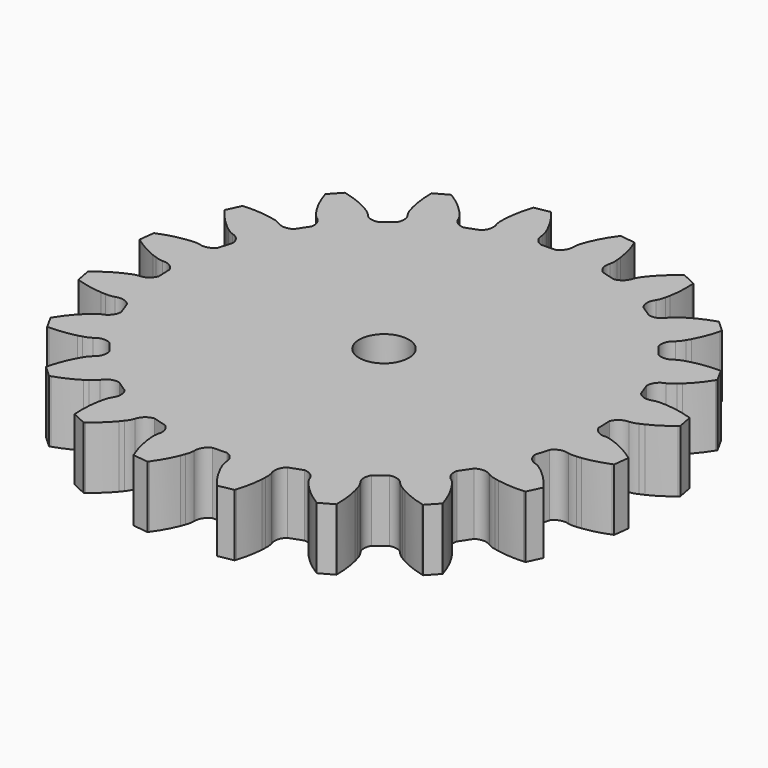
from build123d import *

# Parameters (mm, degrees)
F0_R     = 2
F1_DEPTH = 5


# Not quite as in the source:
# - ends of sketch curves that miss each other by under 0.0002 mm in the source are joined


with BuildPart() as f1:
    # F0 (on Top) → F1 (new body)
    with BuildSketch(Plane.XY):
        with BuildLine():
            ThreePointArc((6.2795421224, 17.2528949711), (5.9372089952, 16.6897816616), (5.3292660269, 16.4354316735))
            Line((5.3292660269, 16.4354316735), (4.238829, 16.749832))
            ThreePointArc((4.238829, 16.749832), (3.8596188728, 17.2887997141), (3.8696296081, 17.947730134))
            ThreePointArc((3.8696296081, 17.947730134), (3.9098326338, 18.2899811197), (3.8900979523, 18.6340169931))
            Line((3.8900979523, 18.6340169931), (3.85527, 18.998924))
            ThreePointArc((3.85527, 18.998924), (3.6466807278, 20.0297301014), (3.312523712, 21.0269318832))
            Line((3.312523712, 21.0269318832), (3.259754, 21.158733))
            Line((3.259754, 21.158733), (2.017975, 21.313043))
            Line((2.017975, 21.313043), (1.934553, 21.198166))
            ThreePointArc((1.934553, 21.198166), (1.3664960287, 20.3130778427), (0.9119624977, 19.3646732036))
            Line((0.9119624977, 19.3646732036), (0.78888, 19.019387))
            ThreePointArc((0.78888, 19.019387), (0.6855432602, 18.6906435099), (0.6407608463, 18.3489640066))
            ThreePointArc((0.6407608463, 18.3489640066), (0.4891935662, 17.707625921), (-0.0103961103, 17.2778602637))
            Line((-0.0103961103, 17.2778602637), (-1.144616, 17.239907))
            ThreePointArc((-1.144616, 17.239907), (-1.6718177114, 17.6353149503), (-1.8659179767, 18.2650879996))
            ThreePointArc((-1.8659179767, 18.2650879996), (-1.9334407464, 18.6030096473), (-2.0585228, 18.9241090987))
            Line((-2.0585228, 18.9241090987), (-2.204412, 19.260394))
            ThreePointArc((-2.204412, 19.260394), (-2.7213270618, 20.1762961465), (-3.3472816933, 21.021431258))
            Line((-3.3472816933, 21.021431258), (-3.438197, 21.130471))
            Line((-3.438197, 21.130471), (-4.666884, 20.893497))
            Line((-4.666884, 20.893497), (-4.710725, 20.758465))
            ThreePointArc((-4.710725, 20.758465), (-4.9774723389, 19.7411552057), (-5.1166863028, 18.6987100215))
            Line((-5.1166863028, 18.6987100215), (-5.127045, 18.332291))
            ThreePointArc((-5.127045, 18.332291), (-5.1237362452, 17.9877011205), (-5.0607420433, 17.648905988))
            ThreePointArc((-5.0607420433, 17.648905988), (-5.0067049946, 16.9921224763), (-5.3490383291, 16.4290093826))
            Line((-5.3490383291, 16.4290093826), (-6.416021, 16.04242))
            ThreePointArc((-6.416021, 16.04242), (-7.0396053696, 16.2555600272), (-7.4188161099, 16.7945296579))
            ThreePointArc((-7.4188161099, 16.7945296579), (-7.5874575289, 17.0950469339), (-7.805642719, 17.361778299))
            Line((-7.805642719, 17.361778299), (-8.04831, 17.636525))
            ThreePointArc((-8.04831, 17.636525), (-8.822951725, 18.3478589308), (-9.6794307515, 18.9581993988))
            Line((-9.6794307515, 18.9581993988), (-9.799595, 19.033811))
            Line((-9.799595, 19.033811), (-10.894916, 18.428749))
            Line((-10.894916, 18.428749), (-10.894883, 18.286778))
            ThreePointArc((-10.894883, 18.286778), (-10.8342091412, 17.2368317381), (-10.6444761882, 16.2023879533))
            Line((-10.6444761882, 16.2023879533), (-10.541097, 15.850697))
            ThreePointArc((-10.541097, 15.850697), (-10.4314703301, 15.5240012928), (-10.2668657315, 15.2212541779))
            ThreePointArc((-10.2668657315, 15.2212541779), (-10.0125146027, 14.6133081664), (-10.1640812817, 13.9719691712))
            Line((-10.1640812817, 13.9719691712), (-11.059377, 13.274587))
            ThreePointArc((-11.059377, 13.274587), (-11.7183065515, 13.284596409), (-12.2455078303, 13.6800041194))
            ThreePointArc((-12.2455078303, 13.6800041194), (-12.4987620125, 13.9137031189), (-12.7886931291, 14.0999567544))
            Line((-12.7886931291, 14.0999567544), (-13.104382, 14.286265))
            ThreePointArc((-13.104382, 14.286265), (-14.0609263803, 14.723407966), (-15.0640920585, 15.0392097641))
            Line((-15.0640920585, 15.0392097641), (-15.20174, 15.073991))
            Line((-15.20174, 15.073991), (-16.056476, 14.16007))
            Line((-16.056476, 14.16007), (-16.012575, 14.025056))
            ThreePointArc((-16.012575, 14.025056), (-15.6304195227, 13.0452436642), (-15.1303121532, 12.1200599045))
            Line((-15.1303121532, 12.1200599045), (-14.923314, 11.817531))
            ThreePointArc((-14.923314, 11.817531), (-14.7180959918, 11.5407024212), (-14.4679937608, 11.303638301))
            ThreePointArc((-14.4679937608, 11.303638301), (-14.0382262447, 10.8040458442), (-13.9841899305, 10.1472587473))
            Line((-13.9841899305, 10.1472587473), (-14.620166, 9.207347))
            ThreePointArc((-14.620166, 9.207347), (-15.2499383725, 9.0132480289), (-15.87352412, 9.22638884))
            ThreePointArc((-15.87352412, 9.22638884), (-16.1865976161, 9.3703858687), (-16.5198940041, 9.4579299761))
            Line((-16.5198940041, 9.4579299761), (-16.877707, 9.537571))
            ThreePointArc((-16.877707, 9.537571), (-17.9225197597, 9.657729375), (-18.9741749647, 9.6480795034))
            Line((-18.9741749647, 9.6480795034), (-19.115832, 9.638622))
            Line((-19.115832, 9.638622), (-19.646318, 8.5053))
            Line((-19.646318, 8.5053), (-19.562844, 8.390465))
            ThreePointArc((-19.562844, 8.390465), (-18.8966142395, 7.5766989313), (-18.1350863391, 6.8513385968))
            Line((-18.1350863391, 6.8513385968), (-17.844734, 6.627582))
            ThreePointArc((-17.844734, 6.627582), (-17.5640125021, 6.4277153406), (-17.2528940551, 6.2795398526))
            ThreePointArc((-17.2528940551, 6.2795398526), (-16.6897826616, 5.9372089952), (-16.4354326735, 5.3292660269))
            Line((-16.4354326735, 5.3292660269), (-16.74983, 4.238829))
            ThreePointArc((-16.74983, 4.238829), (-17.2888002619, 3.8596190122), (-17.9477302386, 3.869629302))
            ThreePointArc((-17.9477302386, 3.869629302), (-18.2899776143, 3.9098326485), (-18.6340139723, 3.8900978098))
            Line((-18.6340139723, 3.8900978098), (-18.998923, 3.85527))
            ThreePointArc((-18.998923, 3.85527), (-20.0297311014, 3.6466807278), (-21.0269328832, 3.312523712))
            Line((-21.0269328832, 3.312523712), (-21.158733, 3.259754))
            Line((-21.158733, 3.259754), (-21.313042, 2.017975))
            Line((-21.313042, 2.017975), (-21.198166, 1.934553))
            ThreePointArc((-21.198166, 1.934553), (-20.3130761949, 1.3664962251), (-19.3646712036, 0.9119624977))
            Line((-19.3646712036, 0.9119624977), (-19.019386, 0.78888))
            ThreePointArc((-19.019386, 0.78888), (-18.6906425099, 0.6855432602), (-18.3489630066, 0.6407608463))
            ThreePointArc((-18.3489630066, 0.6407608463), (-17.7076245117, 0.4891939253), (-17.2778584127, -0.0103957543))
            Line((-17.2778584127, -0.0103957543), (-17.239905, -1.144616))
            ThreePointArc((-17.239905, -1.144616), (-17.6353134914, -1.6718180921), (-18.2650869994, -1.8659179615))
            ThreePointArc((-18.2650869994, -1.8659179615), (-18.6030081703, -1.933440607), (-18.9241080987, -2.0585228))
            Line((-18.9241080987, -2.0585228), (-19.260395, -2.204412))
            ThreePointArc((-19.260395, -2.204412), (-20.1762931465, -2.7213270618), (-21.021428258, -3.3472816933))
            Line((-21.021428258, -3.3472816933), (-21.130471, -3.438197))
            Line((-21.130471, -3.438197), (-20.893497, -4.666884))
            Line((-20.893497, -4.666884), (-20.758464, -4.710725))
            ThreePointArc((-20.758464, -4.710725), (-19.7411532504, -4.9774725271), (-18.6987080265, -5.1166863735))
            Line((-18.6987080265, -5.1166863735), (-18.332287, -5.127045))
            ThreePointArc((-18.332287, -5.127045), (-17.9877021205, -5.1237362452), (-17.648906988, -5.0607420433))
            ThreePointArc((-17.648906988, -5.0607420433), (-16.9921192426, -5.0067048135), (-16.4290058079, -5.3490378347))
            Line((-16.4290058079, -5.3490378347), (-16.042417, -6.416021))
            ThreePointArc((-16.042417, -6.416021), (-16.2555580318, -7.0396053757), (-16.7945276579, -7.4188161099))
            ThreePointArc((-16.7945276579, -7.4188161099), (-17.0950436381, -7.5874573272), (-17.3617747863, -7.8056422191))
            Line((-17.3617747863, -7.8056422191), (-17.636522, -8.04831))
            ThreePointArc((-17.636522, -8.04831), (-18.3478589308, -8.822951725), (-18.9581993988, -9.6794307515))
            Line((-18.9581993988, -9.6794307515), (-19.03381, -9.799595))
            Line((-19.03381, -9.799595), (-18.42875, -10.894916))
            Line((-18.42875, -10.894916), (-18.286777, -10.894883))
            ThreePointArc((-18.286777, -10.894883), (-17.2368287381, -10.8342091412), (-16.2023849533, -10.6444761882))
            Line((-16.2023849533, -10.6444761882), (-15.850698, -10.541097))
            ThreePointArc((-15.850698, -10.541097), (-15.5239982928, -10.4314703301), (-15.2212511779, -10.2668657315))
            ThreePointArc((-15.2212511779, -10.2668657315), (-14.61330897, -10.0125146688), (-13.9719699014, -10.1640808378))
            Line((-13.9719699014, -10.1640808378), (-13.274586, -11.059377))
            ThreePointArc((-13.274586, -11.059377), (-13.2845965413, -11.7183069384), (-13.6800047882, -12.245508301))
            ThreePointArc((-13.6800047882, -12.245508301), (-13.9137001189, -12.4987620125), (-14.0999537544, -12.7886931291))
            Line((-14.0999537544, -12.7886931291), (-14.286265, -13.104382))
            ThreePointArc((-14.286265, -13.104382), (-14.723406966, -14.0609263803), (-15.0392087641, -15.0640920585))
            Line((-15.0392087641, -15.0640920585), (-15.073988, -15.20174))
            Line((-15.073988, -15.20174), (-14.160067, -16.056476))
            Line((-14.160067, -16.056476), (-14.025055, -16.012575))
            ThreePointArc((-14.025055, -16.012575), (-13.0452438471, -15.6304191443), (-12.1200601843, -15.1303117043))
            Line((-12.1200601843, -15.1303117043), (-11.81753, -14.923314))
            ThreePointArc((-11.81753, -14.923314), (-11.5406986541, -14.7180961981), (-11.3036346881, -14.4679942479))
            ThreePointArc((-11.3036346881, -14.4679942479), (-10.8040460838, -14.038226345), (-10.1472587473, -13.9841899305))
            Line((-10.1472587473, -13.9841899305), (-9.207345, -14.620166))
            ThreePointArc((-9.207345, -14.620166), (-9.0132460291, -15.2499383848), (-9.2263872, -15.8735246))
            ThreePointArc((-9.2263872, -15.8735246), (-9.3703848687, -16.1865976161), (-9.4579289761, -16.5198940041))
            Line((-9.4579289761, -16.5198940041), (-9.537568, -16.877707))
            ThreePointArc((-9.537568, -16.877707), (-9.6577283769, -17.9225197951), (-9.6480784984, -18.9741750354))
            Line((-9.6480784984, -18.9741750354), (-9.638618, -19.115832))
            Line((-9.638618, -19.115832), (-8.505301, -19.646318))
            Line((-8.505301, -19.646318), (-8.390464, -19.562844))
            ThreePointArc((-8.390464, -19.562844), (-7.5766996953, -18.8966140207), (-6.8513391825, -18.1350858465))
            Line((-6.8513391825, -18.1350858465), (-6.62758, -17.844734))
            ThreePointArc((-6.62758, -17.844734), (-6.4277133406, -17.5640125021), (-6.2795378526, -17.2528940551))
            ThreePointArc((-6.2795378526, -17.2528940551), (-5.9372079952, -16.6897826616), (-5.3292650269, -16.4354326735))
            Line((-5.3292650269, -16.4354326735), (-4.238828, -16.74983))
            ThreePointArc((-4.238828, -16.74983), (-3.859617942, -17.2888004896), (-3.8696281974, -17.9477299325))
            ThreePointArc((-3.8696281974, -17.9477299325), (-3.9098316455, -18.289977513), (-3.8900968098, -18.6340139723))
            Line((-3.8900968098, -18.6340139723), (-3.855269, -18.998923))
            ThreePointArc((-3.855269, -18.998923), (-3.6466796615, -20.0297313492), (-3.3125225708, -21.0269332314))
            Line((-3.3125225708, -21.0269332314), (-3.259753, -21.158733))
            Line((-3.259753, -21.158733), (-2.017974, -21.313042))
            Line((-2.017974, -21.313042), (-1.934552, -21.198166))
            ThreePointArc((-1.934552, -21.198166), (-1.3664951336, -20.3130760309), (-0.9119613566, -19.3646708554))
            Line((-0.9119613566, -19.3646708554), (-0.788879, -19.019386))
            ThreePointArc((-0.788879, -19.019386), (-0.6855422602, -18.6906425099), (-0.6407598463, -18.3489630066))
            ThreePointArc((-0.6407598463, -18.3489630066), (-0.4891926857, -17.7076241175), (0.0103976053, -17.2778580567))
            Line((0.0103976053, -17.2778580567), (1.144617, -17.239905))
            ThreePointArc((1.144617, -17.239905), (1.6718193644, -17.6353138784), (1.8659189615, -18.2650869994))
            ThreePointArc((1.8659189615, -18.2650869994), (1.9334425295, -18.6030079051), (2.0585246041, -18.9241077018))
            Line((2.0585246041, -18.9241077018), (2.204413, -19.260395))
            ThreePointArc((2.204413, -19.260395), (2.7213287677, -20.1762926934), (3.347283279, -21.0214277654))
            Line((3.347283279, -21.0214277654), (3.438198, -21.130471))
            Line((3.438198, -21.130471), (4.666886, -20.893497))
            Line((4.666886, -20.893497), (4.710727, -20.758464))
            ThreePointArc((4.710727, -20.758464), (4.9774735574, -19.7411530969), (5.1166873735, -18.6987080265))
            Line((5.1166873735, -18.6987080265), (5.127046, -18.332287))
            ThreePointArc((5.127046, -18.332287), (5.1237372415, -17.9877020819), (5.0607430433, -17.648906988))
            ThreePointArc((5.0607430433, -17.648906988), (5.0067057691, -16.9921194304), (5.3490388347, -16.4290058079))
            Line((5.3490388347, -16.4290058079), (6.416022, -16.042417))
            ThreePointArc((6.416022, -16.042417), (7.0396064935, -16.2555581202), (7.4188171966, -16.7945279394))
            ThreePointArc((7.4188171966, -16.7945279394), (7.5874585239, -17.0950439265), (7.8056437065, -17.3617752862))
            Line((7.8056437065, -17.3617752862), (8.048311, -17.636522))
            ThreePointArc((8.048311, -17.636522), (8.8229534556, -18.3478587126), (9.6794327515, -18.9581993988))
            Line((9.6794327515, -18.9581993988), (9.799594, -19.03381))
            Line((9.799594, -19.03381), (10.894917, -18.42875))
            Line((10.894917, -18.42875), (10.894884, -18.286777))
            ThreePointArc((10.894884, -18.286777), (10.8342111412, -17.2368287381), (10.6444781882, -16.2023849533))
            Line((10.6444781882, -16.2023849533), (10.541099, -15.850698))
            ThreePointArc((10.541099, -15.850698), (10.4314713301, -15.5239982928), (10.2668667315, -15.2212511779))
            ThreePointArc((10.2668667315, -15.2212511779), (10.0125156955, -14.613309295), (10.1640818378, -13.9719699014))
            Line((10.1640818378, -13.9719699014), (11.059379, -13.274586))
            ThreePointArc((11.059379, -13.274586), (11.7183099384, -13.2845965413), (12.245511301, -13.6800047882))
            ThreePointArc((12.245511301, -13.6800047882), (12.4987616623, -13.9136998482), (12.7886923455, -14.0999533426))
            Line((12.7886923455, -14.0999533426), (13.104383, -14.286265))
            ThreePointArc((13.104383, -14.286265), (14.060930245, -14.7234072983), (15.0640960005, -15.0392089978))
            Line((15.0640960005, -15.0392089978), (15.201741, -15.073988))
            Line((15.201741, -15.073988), (16.056479, -14.160067))
            Line((16.056479, -14.160067), (16.012574, -14.025055))
            ThreePointArc((16.012574, -14.025055), (15.6304210332, -13.0452436071), (15.1303134245, -12.1200597354))
            Line((15.1303134245, -12.1200597354), (14.923317, -11.81753))
            ThreePointArc((14.923317, -11.81753), (14.7180980246, -11.5406984582), (14.4679962479, -11.3036346881))
            ThreePointArc((14.4679962479, -11.3036346881), (14.0382282244, -10.8040457957), (13.9841918776, -10.1472589711))
            Line((13.9841918776, -10.1472589711), (14.620167, -9.207345))
            ThreePointArc((14.620167, -9.207345), (15.2499397847, -9.0132460352), (15.87352624, -9.22638768))
            ThreePointArc((15.87352624, -9.22638768), (16.1866007432, -9.3703845561), (16.5198970326, -9.4579288096))
            Line((16.5198970326, -9.4579288096), (16.877707, -9.537568))
            ThreePointArc((16.877707, -9.537568), (17.9225212931, -9.6577284031), (18.9741770304, -9.6480784276))
            Line((18.9741770304, -9.6480784276), (19.115831, -9.638618))
            Line((19.115831, -9.638618), (19.646322, -8.505301))
            Line((19.646322, -8.505301), (19.562846, -8.390464))
            ThreePointArc((19.562846, -8.390464), (18.8966178219, -7.5766994811), (18.1350898465, -6.8513391825))
            Line((18.1350898465, -6.8513391825), (17.844734, -6.62758))
            ThreePointArc((17.844734, -6.62758), (17.5640139059, -6.427713578), (17.2528959327, -6.2795381803))
            ThreePointArc((17.2528959327, -6.2795381803), (16.6897816616, -5.9372079952), (16.4354316735, -5.3292650269))
            Line((16.4354316735, -5.3292650269), (16.749832, -4.238828))
            ThreePointArc((16.749832, -4.238828), (17.2887999418, -3.8596178026), (17.9477298279, -3.8696285035))
            ThreePointArc((17.9477298279, -3.8696285035), (18.2899810184, -3.9098316307), (18.6340169931, -3.8900969523))
            Line((18.6340169931, -3.8900969523), (18.998924, -3.855269))
            ThreePointArc((18.998924, -3.855269), (20.0297303492, -3.6466796615), (21.0269322314, -3.3125225708))
            Line((21.0269322314, -3.3125225708), (21.158733, -3.259753))
            Line((21.158733, -3.259753), (21.313043, -2.017974))
            Line((21.313043, -2.017974), (21.198166, -1.934552))
            ThreePointArc((21.198166, -1.934552), (20.3130776786, -1.3664949372), (19.3646728554, -0.9119613566))
            Line((19.3646728554, -0.9119613566), (19.019387, -0.788879))
            ThreePointArc((19.019387, -0.788879), (18.6906435099, -0.6855422602), (18.3489640066, -0.6407598463))
            ThreePointArc((18.3489640066, -0.6407598463), (17.7076255268, -0.4891923266), (17.2778599077, 0.0103979614))
            Line((17.2778599077, 0.0103979614), (17.239907, 1.144617))
            ThreePointArc((17.239907, 1.144617), (17.6353153373, 1.6718189836), (18.2650879996, 1.8659189767))
            ThreePointArc((18.2650879996, 1.8659189767), (18.6030093821, 1.9334426689), (18.9241087018, 2.0585246041))
            Line((18.9241087018, 2.0585246041), (19.260394, 2.204413))
            ThreePointArc((19.260394, 2.204413), (20.1762956934, 2.7213287677), (21.0214307654, 3.347283279))
            Line((21.0214307654, 3.347283279), (21.130471, 3.438198))
            Line((21.130471, 3.438198), (20.893497, 4.666886))
            Line((20.893497, 4.666886), (20.758465, 4.710727))
            ThreePointArc((20.758465, 4.710727), (19.7411550522, 4.9774733691), (18.6987100215, 5.1166873028))
            Line((18.6987100215, 5.1166873028), (18.332291, 5.127046))
            ThreePointArc((18.332291, 5.127046), (17.9877010819, 5.1237372415), (17.648905988, 5.0607430433))
            ThreePointArc((17.648905988, 5.0607430433), (16.9921226641, 5.0067059502), (16.4290093826, 5.3490393291))
            Line((16.4290093826, 5.3490393291), (16.04242, 6.416022))
            ThreePointArc((16.04242, 6.416022), (16.2555601156, 7.0396064874), (16.7945299394, 7.4188171966))
            ThreePointArc((16.7945299394, 7.4188171966), (17.0950472222, 7.5874587256), (17.3617787988, 7.8056442063))
            Line((17.3617787988, 7.8056442063), (17.636525, 8.048311))
            ThreePointArc((17.636525, 8.048311), (18.3478587126, 8.8229534556), (18.9581993988, 9.6794327515))
            Line((18.9581993988, 9.6794327515), (19.033811, 9.799594))
            Line((19.033811, 9.799594), (18.428749, 10.894917))
            Line((18.428749, 10.894917), (18.286778, 10.894884))
            ThreePointArc((18.286778, 10.894884), (17.2368317381, 10.8342111412), (16.2023879533, 10.6444781882))
            Line((16.2023879533, 10.6444781882), (15.850697, 10.541099))
            ThreePointArc((15.850697, 10.541099), (15.5240012928, 10.4314713301), (15.2212541779, 10.2668667315))
            ThreePointArc((15.2212541779, 10.2668667315), (14.6133084914, 10.0125156294), (13.9719691712, 10.1640822817))
            Line((13.9719691712, 10.1640822817), (13.274587, 11.059379))
            ThreePointArc((13.274587, 11.059379), (13.284596409, 11.7183095515), (13.6800041194, 12.2455108303))
            ThreePointArc((13.6800041194, 12.2455108303), (13.9137028482, 12.4987616623), (14.0999563426, 12.7886923455))
            Line((14.0999563426, 12.7886923455), (14.286265, 13.104383))
            ThreePointArc((14.286265, 13.104383), (14.7234082983, 14.060930245), (15.0392099978, 15.0640960005))
            Line((15.0392099978, 15.0640960005), (15.073991, 15.201741))
            Line((15.073991, 15.201741), (14.16007, 16.056479))
            Line((14.16007, 16.056479), (14.025056, 16.012574))
            ThreePointArc((14.025056, 16.012574), (13.0452434242, 15.6304214116), (12.1200594556, 15.1303138734))
            Line((12.1200594556, 15.1303138734), (11.817531, 14.923317))
            ThreePointArc((11.817531, 14.923317), (11.5407022254, 14.7180978183), (11.303638301, 14.4679957608))
            ThreePointArc((11.303638301, 14.4679957608), (10.8040455561, 14.0382281242), (10.1472589711, 13.9841918776))
            Line((10.1472589711, 13.9841918776), (9.207347, 14.620167))
            ThreePointArc((9.207347, 14.620167), (9.013248035, 15.2499397725), (9.22638932, 15.87352576))
            ThreePointArc((9.22638932, 15.87352576), (9.3703855561, 16.1866007432), (9.4579298096, 16.5198970326))
            Line((9.4579298096, 16.5198970326), (9.537571, 16.877707))
            ThreePointArc((9.537571, 16.877707), (9.6577294013, 17.9225212577), (9.6480794326, 18.9741769596))
            Line((9.6480794326, 18.9741769596), (9.638622, 19.115831))
            Line((9.638622, 19.115831), (8.5053, 19.646322))
            Line((8.5053, 19.646322), (8.390465, 19.562846))
            ThreePointArc((8.390465, 19.562846), (7.576698717, 18.8966180408), (6.8513385968, 18.1350903391))
            Line((6.8513385968, 18.1350903391), (6.627582, 17.844734))
            ThreePointArc((6.627582, 17.844734), (6.427715578, 17.5640139059), (6.2795421224, 17.2528949711))
        make_face()
        with Locations((2e-06, 2e-06)):
            Circle(F0_R, mode=Mode.SUBTRACT)
    extrude(amount=F1_DEPTH)


solid = f1.part
